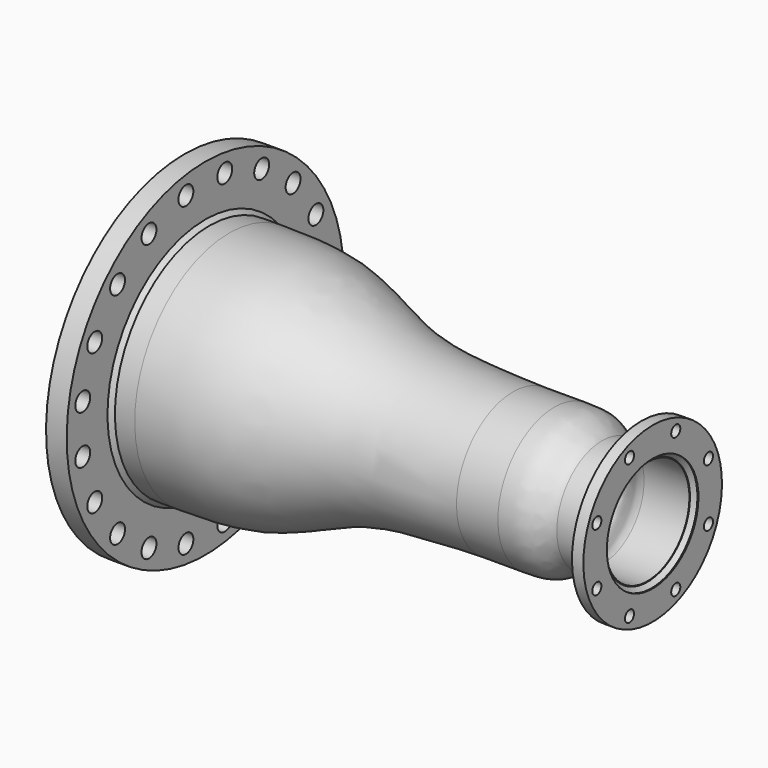
from build123d import *

# Parameters (mm, degrees)
F5_D      = 36
F5_DEPTH  = 50
F5_TIP    = 10.8154911425
F10_D     = 22
F10_DEPTH = 50
F10_TIP   = 6.6094668093


# Not quite as in the source:
# - a feature names something its author has since deleted; it is built from what else it names


with BuildPart() as f1:
    # F0 (on Front) → F1 (revolve)
    with BuildSketch(Plane.XZ):
        Polygon((-337.6619696266, 230), (-329.6619696266, 230), (-299.6619696266, 230), (-299.6619696266, 236.5), (-299.6619696266, 335), (-339.6619696266, 335), (-339.6619696266, 230), align=None)
    revolve(axis=Axis((45.028969672, 0, 0), (1, 0, 0)))

    # F5
    with Locations(Plane(origin=(-339.6619696266, 0, 0), x_dir=(0, -1, 0), z_dir=(-1, 0, 0))):
        with Locations((-46.9303395121, 296.3065021785), (46.9303395121, 296.3065021785), (136.1971499219, 267.3019572565), (212.132034356, 212.132034356), (267.3019572565, 136.1971499219), (296.3065021785, 46.9303395121), (296.3065021785, -46.9303395121), (267.3019572565, -136.1971499219), (212.132034356, -212.132034356), (136.1971499219, -267.3019572565), (46.9303395121, -296.3065021785), (-136.1971499219, -267.3019572565), (-212.132034356, -212.132034356), (-267.3019572565, -136.1971499219), (-296.3065021785, -46.9303395121), (-46.9303395121, -296.3065021785), (-296.3065021785, 46.9303395121), (-267.3019572565, 136.1971499219), (-212.132034356, 212.132034356), (-136.1971499219, 267.3019572565)):
            Hole(F5_D / 2, depth=F5_DEPTH)
            with Locations((0, 0, -(F5_DEPTH + F5_TIP / 2))):  # 118° drill point
                Cone(0, F5_D / 2, F5_TIP, mode=Mode.SUBTRACT)


with BuildPart() as f2:
    # F0 (on Front) → F2 (revolve)
    with BuildSketch(Plane.XZ):
        with BuildLine():
            add(Edge.make_bspline(
                [(-253.3748149872, 228.5), (-207.6811939478, 228.0596494675), (-107.9575658009, 229.4268890138), (23.480264241, 163.9475460602), (130.3051072184, 141.5938575123), (236.1741111698, 137.8832627127), (295.3158915043, 136.55)],
                knots=[0, 0, 0, 0, 0.2542116463, 0.5070615956, 0.7273664746, 1, 1, 1, 1], degree=3))
            Line((-253.3748149872, 228.5), (-253.4206936962, 218.97))
            add(Edge.make_bspline(
                [(-253.4206936962, 218.97), (-240.2009376391, 219.1843285332), (-206.9350282777, 219.7236602371), (-104.4913953456, 213.6592114843), (23.6305209991, 152.5518060653), (127.1706610346, 134.9560944534), (235.1658650843, 127.3504382511), (277.3244460023, 127.1188372265), (295.3158915043, 127.02)],
                knots=[0, 0, 0, 0, 0.1161918754, 0.2923827322, 0.5019993241, 0.6847543592, 0.8654668957, 1, 1, 1, 1], degree=3))
            Line((295.3158915043, 127.02), (375.3380303734, 127.02))
            Line((375.3380303734, 127.02), (375.3380303734, 136.55))
            Line((375.3380303734, 136.55), (295.3158915043, 136.55))
        make_face()
        Polygon((-299.6619696266, 228.5), (-329.6619696266, 228.5), (-329.6619696266, 222), (-329.6619696266, 218.97), (-253.4206936962, 218.97), (-253.3748149872, 228.5), (-291.6619696266, 228.5), align=None)
    revolve(axis=Axis((45.028969672, 0, 0), (1, 0, 0)))

    # F0 (on Front) → F6 (revolve)
    with BuildSketch(Plane.XZ):
        Polygon((535.3380303734, 109.55), (467.6481485367, 109.55), (467.6481485367, 101.37), (555.3380303734, 101.37), (555.3380303734, 102.7), (555.3380303734, 109.55), (543.3380303734, 109.55), align=None)
        with BuildLine():
            add(Edge.make_bspline(
                [(375.3380303734, 136.55), (389.7872619021, 136.5271284103), (415.2423562214, 135.9865060076), (432.0466082032, 126.8445897583), (450.2065197701, 115.5504833836), (455.557771098, 110.3991705165), (467.6481485367, 109.55)],
                knots=[0, 0, 0, 0, 0.3238691381, 0.547454705, 0.7678911056, 1, 1, 1, 1], degree=3))
            Line((375.3380303734, 136.55), (375.3380303734, 127.02))
            add(Edge.make_bspline(
                [(375.3380303734, 127.02), (379.6535656436, 127.1019095607), (389.5057717451, 127.2889060336), (413.704138146, 125.7169560852), (425.9979727104, 119.8448667946), (443.8440547181, 108.4181927763), (455.7879394789, 101.8271287701), (463.8193095231, 101.5175751785), (467.6481485367, 101.37)],
                knots=[0, 0, 0, 0, 0.1572530342, 0.3590028132, 0.5159763971, 0.7055400439, 0.8596204929, 1, 1, 1, 1], degree=3))
            Line((467.6481485367, 101.37), (467.6481485367, 109.55))
        make_face()
    revolve(axis=Axis((45.028969672, 0, 0), (1, 0, 0)))


with BuildPart() as f3:
    # F0 (on Front) → F3 (revolve)
    with BuildSketch(Plane.XZ):
        Polygon((-329.6619696266, 222), (-329.6619696266, 228.5), (-329.6619696266, 230), (-337.6619696266, 230), align=None)
    revolve(axis=Axis((45.028969672, 0, 0), (1, 0, 0)))


with BuildPart() as f3b:
    # F0 (on Front) → F3, piece 2 (revolve)
    with BuildSketch(Plane.XZ):
        Polygon((-299.6619696266, 230), (-299.6619696266, 228.5), (-291.6619696266, 228.5), (-299.6619696266, 236.5), align=None)
    revolve(axis=Axis((45.028969672, 0, 0), (1, 0, 0)))


with BuildPart() as f7:
    # F0 (on Front) → F7 (revolve)
    with BuildSketch(Plane.XZ):
        Polygon((543.3380303734, 167.5), (543.3380303734, 117.55), (543.3380303734, 110.7), (555.3380303734, 110.7), (563.3380303734, 110.7), (565.3380303734, 110.7), (565.3380303734, 167.5), align=None)
    revolve(axis=Axis((45.028969672, 0, 0), (1, 0, 0)))

    # F10
    with Locations(Plane.YZ.offset(565.3380303734)):
        with Locations((134.8864117466, 55.8717811253), (134.8864117466, -55.8717811253), (55.8717811253, -134.8864117466), (-55.8717811253, -134.8864117466), (-134.8864117466, -55.8717811253), (-134.8864117466, 55.8717811253), (-55.8717811253, 134.8864117466), (55.8717811253, 134.8864117466)):
            Hole(F10_D / 2, depth=F10_DEPTH)
            with Locations((0, 0, -(F10_DEPTH + F10_TIP / 2))):  # 118° drill point
                Cone(0, F10_D / 2, F10_TIP, mode=Mode.SUBTRACT)


with BuildPart() as f8:
    # F0 (on Front) → F8 (revolve)
    with BuildSketch(Plane.XZ):
        Polygon((543.3380303734, 117.55), (535.3380303734, 109.55), (543.3380303734, 109.55), (543.3380303734, 110.7), align=None)
    revolve(axis=Axis((45.028969672, 0, 0), (1, 0, 0)))


with BuildPart() as f8b:
    # F0 (on Front) → F8, piece 2 (revolve)
    with BuildSketch(Plane.XZ):
        Polygon((555.3380303734, 109.55), (555.3380303734, 102.7), (563.3380303734, 110.7), (555.3380303734, 110.7), align=None)
    revolve(axis=Axis((45.028969672, 0, 0), (1, 0, 0)))


solid = Compound([f1.part, f2.part, f3.part, f3b.part, f7.part, f8.part, f8b.part])
